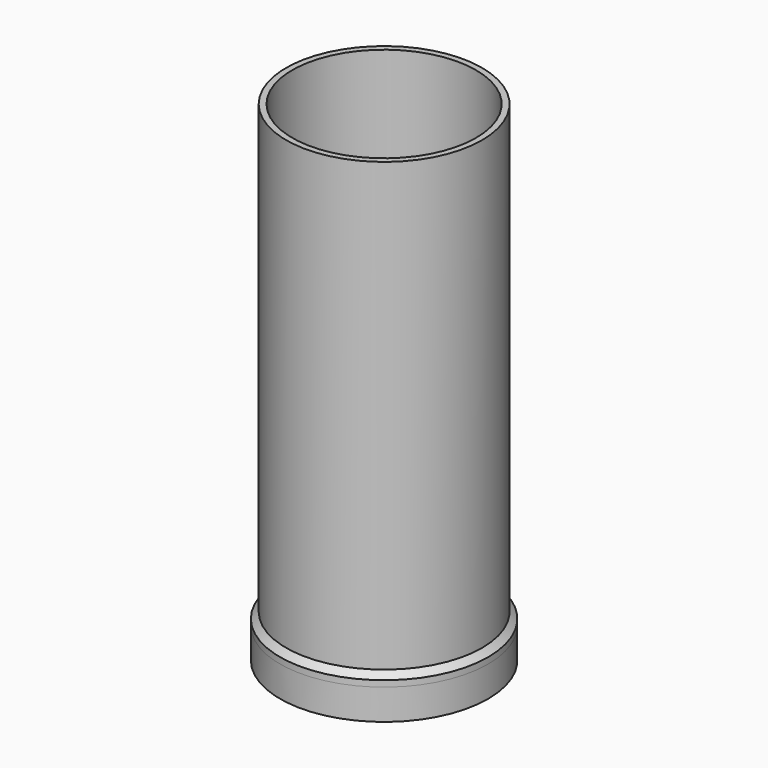
from build123d import *

# Parameters (mm, degrees)
F0_R     = 16
F0_R_2   = 15
F1_DEPTH = 75
F2_R     = 17
F2_R_2   = 16
F3_DEPTH = 5
F4_DEPTH = 2
F5_SIZE  = 0.99999
F6_SIZE  = 0.99999


# Not quite as in the source:
# - a fillet or chamfer is up to 0.001 mm smaller than in the source, because OpenCascade refuses the exact size


with BuildPart() as f1:
    # F0 (on Top) → F1 (new body)
    with BuildSketch(Plane.XY):
        Circle(F0_R)
        Circle(F0_R_2, mode=Mode.SUBTRACT)
    extrude(amount=-F1_DEPTH)

    # F5 (size 1 in the source; OpenCascade refuses exactly that, so slightly less here)
    f5_edges = [f1.edges().sort_by_distance(p)[0] for p in [
        (-15, 0, -75),
    ]]
    chamfer(f5_edges, length=F5_SIZE)


with BuildPart() as f3:
    # F2 (on face) → F3 (new body)
    with BuildSketch(Plane(origin=(0, 0, -75), x_dir=(1, 0, 0), z_dir=(0, 0, -1))):
        Circle(F2_R)
        Circle(F2_R_2, mode=Mode.SUBTRACT)
    extrude(amount=F3_DEPTH)


with BuildPart() as f4:
    # F4 (new): a face of the model
    f4_faces = [f3.part.faces().sort_by_distance(p)[0] for p in [
        (-16.5191673888, 0, -75),
    ]]
    extrude(f4_faces, amount=F4_DEPTH)

    # F6 (size 1 in the source; OpenCascade refuses exactly that, so slightly less here)
    f6_edges = [f4.edges().sort_by_distance(p)[0] for p in [
        (-17, 0, -73),
    ]]
    chamfer(f6_edges, length=F6_SIZE)


solid = Compound([f1.part, f3.part, f4.part])
